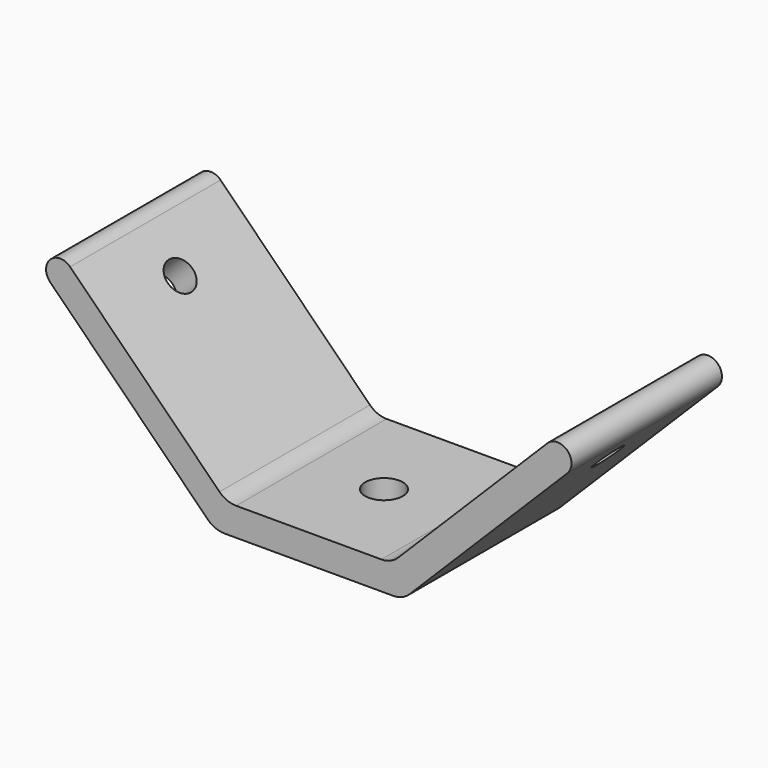
from build123d import *

# Parameters (mm, degrees)
F1_DEPTH = 20
F2_R     = 4
F3_DEPTH = 40.1223203436
F6_D     = 6.6


# Not quite as in the source:
# - a pattern or mirror of a feature is missing from the dataset's text; its kind, count and spacing are read off the source's solid


with BuildPart() as f1:
    # F0 (on Front) → F1 (new body, symmetric)
    with BuildSketch(Plane.XZ):
        with BuildLine():
            Line((-17.9289321881, 0), (0, 0))
            Line((0, 0), (17.9289321881, 0))
            ThreePointArc((17.9289321881, 0), (19.84234935, 0.3806023374), (21.4644660941, 1.4644660941))
            Line((21.4644660941, 1.4644660941), (55, 35))
            ThreePointArc((55, 35), (55, 39.2426406871), (50.7573593129, 39.2426406871))
            Line((50.7573593129, 39.2426406871), (18.9791847198, 7.4644660941))
            ThreePointArc((18.9791847198, 7.4644660941), (17.3570679757, 6.3806023374), (15.4436508139, 6))
            Line((15.4436508139, 6), (0, 6))
            Line((0, 6), (-15.4436508139, 6))
            ThreePointArc((-15.4436508139, 6), (-17.3570679757, 6.3806023374), (-18.9791847198, 7.4644660941))
            Line((-18.9791847198, 7.4644660941), (-50.7573593129, 39.2426406871))
            ThreePointArc((-50.7573593129, 39.2426406871), (-55, 39.2426406871), (-55, 35))
            Line((-55, 35), (-21.4644660941, 1.4644660941))
            ThreePointArc((-21.4644660941, 1.4644660941), (-19.84234935, 0.3806023374), (-17.9289321881, 0))
        make_face()
    extrude(amount=F1_DEPTH, both=True)

    # F2 (on Top) → F3 (cut, through all)
    with BuildSketch(Plane.XY):
        Circle(F2_R)
    extrude(amount=F3_DEPTH, mode=Mode.SUBTRACT)

    # F6 (through all)
    with Locations(Plane(origin=(10, 0, -10), x_dir=(0, 1, 0), z_dir=(0.7071067812, 0, -0.7071067812))):
        with Locations((0, 53.1789772213)):
            f6 = Hole(F6_D / 2)

    # F6_copies: F6 across plane
    add(f6.mirror(Plane(origin=(0, 0, 0), x_dir=(0, 0, -1), z_dir=(-1, 0, 0))), mode=Mode.SUBTRACT)


solid = f1.part
